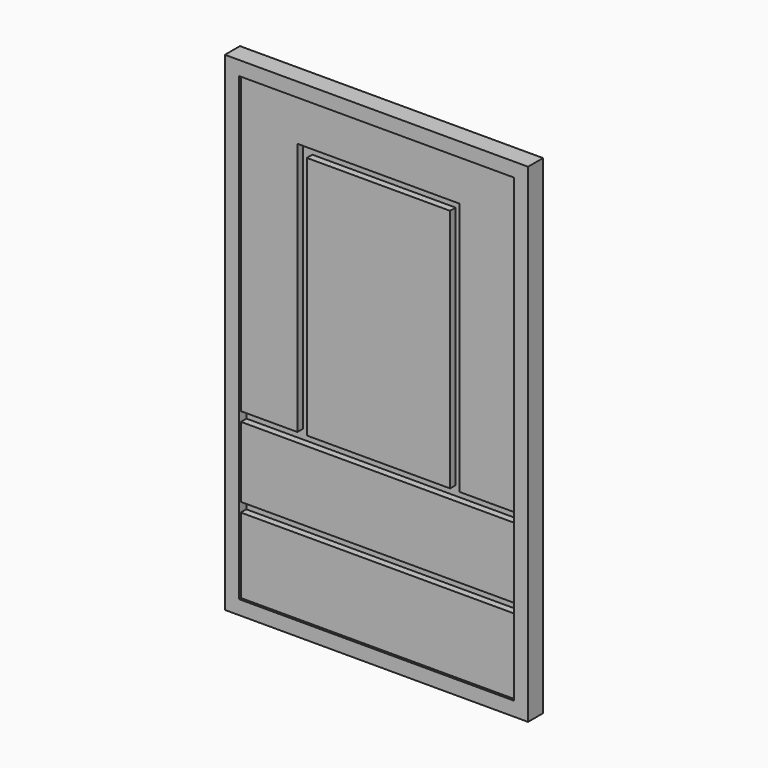
from build123d import *

# Parameters (mm, degrees)
F1_DEPTH      = 12.7
F1_DEPTH_BACK = 12.7
F0_W          = 371.475
F0_H          = 622.3
F2_DEPTH      = 9.398
F2_DEPTH_BACK = 9.398
F3_W          = 193.675
F3_H          = 330.2
F4_DEPTH      = 12.7


# Not quite as in the source:
# - a feature names something its author has since deleted; it is built from what else it names


with BuildPart() as f1:
    # F0 (on Front) → F1 (new body, two sides)
    with BuildSketch(Plane.XZ) as f1_sk:
        Polygon((277.0045676708, 526.3417813361), (648.4795676708, 526.3417813361), (667.5295676708, 545.3917813361), (257.9545676708, 545.3917813361), align=None)
        Polygon((277.0045676708, -95.9582186639), (277.0045676708, 526.3417813361), (257.9545676708, 545.3917813361), (257.9545676708, -115.0082186639), align=None)
        Polygon((667.5295676708, 545.3917813361), (648.4795676708, 526.3417813361), (648.4795676708, -95.9582186639), (667.5295676708, -115.0082186639), align=None)
        Polygon((667.5295676708, -115.0082186639), (648.4795676708, -95.9582186639), (277.0045676708, -95.9582186639), (257.9545676708, -115.0082186639), align=None)
    extrude(amount=-F1_DEPTH)
    extrude(f1_sk.sketch, amount=F1_DEPTH_BACK)

    # F0 (on Front) → F2 (join, two sides)
    with BuildSketch(Plane.XZ) as f2_sk:
        Polygon((667.5295676708, 545.3917813361), (648.4795676708, 526.3417813361), (648.4795676708, -95.9582186639), (667.5295676708, -115.0082186639), align=None)
        Polygon((277.0045676708, 526.3417813361), (648.4795676708, 526.3417813361), (667.5295676708, 545.3917813361), (257.9545676708, 545.3917813361), align=None)
        Polygon((667.5295676708, -115.0082186639), (648.4795676708, -95.9582186639), (277.0045676708, -95.9582186639), (257.9545676708, -115.0082186639), align=None)
        Polygon((277.0045676708, -95.9582186639), (277.0045676708, 526.3417813361), (257.9545676708, 545.3917813361), (257.9545676708, -115.0082186639), align=None)
        with Locations((462.7420676708, 215.1917813361)):
            Rectangle(F0_W, F0_H)
    extrude(amount=F2_DEPTH)
    extrude(f2_sk.sketch, amount=-F2_DEPTH_BACK)

    # F3 (on face) → F4 (cut)
    with BuildSketch(Plane.XZ):
        Polygon((276.66666205, 5.6417813361), (648.4795676708, 5.6417813361), (648.4795676708, 18.3417813361), (277.0045676708, 18.3417813361), align=None)
        Polygon((572.2795676708, 456.4917813361), (572.2795676708, 469.1917813361), (353.2045676708, 469.1917813361), (353.2045676708, 456.4917813361), (353.2045676708, 126.2917813361), (277.0045676708, 126.2917813361), (277.0045676708, 113.5917813361), (648.4795676708, 113.5917813361), (648.4795676708, 126.2917813361), (572.2795676708, 126.2917813361), align=None)
        with Locations((462.7420676708, 291.3917813361)):
            Rectangle(F3_W, F3_H, mode=Mode.SUBTRACT)
    extrude(amount=F4_DEPTH, mode=Mode.SUBTRACT)


solid = f1.part
